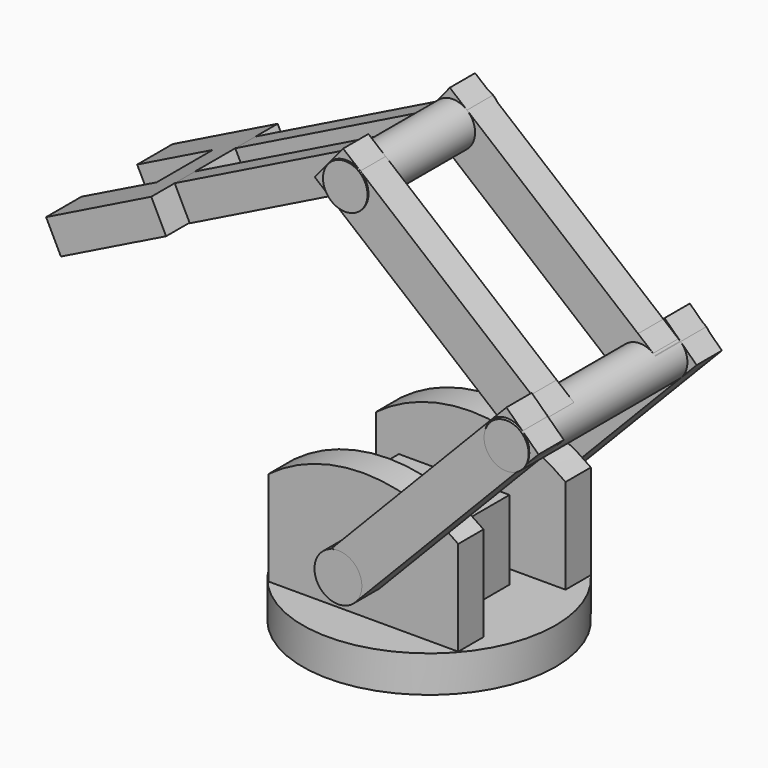
from build123d import *

# Parameters (mm, degrees)
F0_R           = 50.8
F1_DEPTH       = 14.69634
F2_W           = 76.2
F2_H           = 12.7
F3_DEPTH       = 38.1
F5_DEPTH       = 12.7
F7_DEPTH       = 12.7
F8_W           = 44.45
F8_H           = 25.4
F9_DEPTH       = 31.75
F10_R          = 9.525
F11_DEPTH      = 68.24913
F12_R          = 9.525
F13_DEPTH      = 66.70077
F14_R          = 9.525
F15_DEPTH      = 12.7
F16_R          = 9.525
F17_DEPTH      = 12.7
F19_DEPTH      = 12.7
F21_R          = 8.9662
F22_DEPTH      = 79.74323
F22_DEPTH_BACK = 12.92457
F24_DEPTH      = 12.7
F26_R          = 8.9540969
F27_DEPTH      = 54.0361
F27_DEPTH_BACK = 13.11087
F29_DEPTH      = 10.16
F31_W          = 13.2109493386
F31_H          = 63.5
F32_DEPTH      = 13.44194
F34_DEPTH      = 13.41844
F35_W          = 33.9267599266
F35_H          = 17.78
F36_DEPTH      = 13.32265
F37_R          = 8.9662
F38_DEPTH      = 12.7
F39_R          = 8.9662
F40_DEPTH      = 12.7
F41_R          = 8.9540969
F42_DEPTH      = 12.7
F43_R          = 8.9540969
F44_DEPTH      = 12.7


# Not quite as in the source:
# - a feature names something its author has since deleted; it is built from what else it names


with BuildPart() as f1:
    # F0 (on Top) → F1 (new body)
    with BuildSketch(Plane.XY):
        with Locations((78.1534910202, 35.6075726449)):
            Circle(F0_R)
    extrude(amount=F1_DEPTH)

    # F2 (on face) → F3 (join)
    with BuildSketch(Plane.XY.offset(14.69634)):
        with Locations((78.1534910202, 8.9485988323)):
            Rectangle(F2_W, F2_H)
        with Locations((78.1534910202, 62.8586142955)):
            Rectangle(F2_W, F2_H)
    extrude(amount=F3_DEPTH)

    # F4 (on face) → F5 (join)
    with BuildSketch(Plane.XZ.offset(-2.5985988323)):
        with BuildLine():
            Line((40.0534910202, 52.79634), (116.2534910202, 52.79634))
            ThreePointArc((116.2534910202, 52.79634), (78.1534910202, 65.49634), (40.0534910202, 52.79634))
        make_face()
    extrude(amount=-F5_DEPTH)

    # F6 (on face) → F7 (join)
    with BuildSketch(Plane.XZ.offset(-56.5086142955)):
        with BuildLine():
            Line((40.0534910202, 52.79634), (116.2534910202, 52.79634))
            ThreePointArc((116.2534910202, 52.79634), (78.1534910202, 65.49634), (40.0534910202, 52.79634))
        make_face()
    extrude(amount=-F7_DEPTH)

    # F8 (on face) → F9 (join)
    with BuildSketch(Plane.XY.offset(14.69634)):
        with Locations((78.1534910202, 35.4908860509)):
            Rectangle(F8_W, F8_H)
    extrude(amount=F9_DEPTH)

    # F10 (on face) → F11 (cut)
    with BuildSketch(Plane.XZ.offset(-2.5985988323)):
        with Locations((78.1534910202, 33.74634)):
            Circle(F10_R)
    extrude(amount=-F11_DEPTH, mode=Mode.SUBTRACT)


with BuildPart() as f13:
    # F12 (on face) → F13 (new body)
    with BuildSketch(Plane.XZ.offset(-2.5985988323)):
        with Locations((78.1534910202, 33.74634)):
            Circle(F12_R)
    extrude(amount=-F13_DEPTH)

    # F14 (on face) → F15 (join)
    with BuildSketch(Plane.XZ.offset(-2.5985988323)):
        with Locations((78.1534910202, 33.74634)):
            Circle(F14_R)
    extrude(amount=F15_DEPTH)

    # F16 (on face) → F17 (join)
    with BuildSketch(Plane(origin=(0, 69.2993688323, 0), x_dir=(-1, 0, 0), z_dir=(0, 1, 0))):
        with Locations((-78.1534910202, 33.74634)):
            Circle(F16_R)
    extrude(amount=F17_DEPTH)


with BuildPart() as f19:
    # F18 (on face) → F19 (new body)
    with BuildSketch(Plane.XZ.offset(-2.5985988323)):
        with BuildLine():
            Line((145.7822117796, 115.867993462), (94.9363889392, 63.238354479))
            ThreePointArc((94.9363889392, 63.238354479), (103.9505756834, 60.0201318692), (112.3786539474, 55.4836115944))
            Line((112.3786539474, 55.4836115944), (158.6790101463, 103.4083160324))
            Line((158.6790101463, 103.4083160324), (145.7822117796, 115.867993462))
        make_face()
        with BuildLine():
            Line((94.9363889392, 63.238354479), (75.1891385244, 42.7983143305))
            ThreePointArc((75.1891385244, 42.7983143305), (83.7432212229, 41.4587028845), (87.6784910202, 33.74634))
            ThreePointArc((87.6784910202, 33.74634), (87.0779374466, 30.4176944823), (85.3520068243, 27.5087927883))
            Line((85.3520068243, 27.5087927883), (112.3786539474, 55.4836115944))
            ThreePointArc((112.3786539474, 55.4836115944), (103.9505756834, 60.0201318692), (94.9363889392, 63.238354479))
        make_face()
    extrude(amount=F19_DEPTH)


with BuildPart() as f20_1:
    # F20: copy of F19
    add(f19.part.moved(Location((0, 79.43989, -0.67967))))

    # F39 (on face) → F40 (cut)
    with BuildSketch(Plane(origin=(0, 82.0384888323, 0), x_dir=(-1, 0, 0), z_dir=(0, 1, 0))):
        with Locations((-146.0007722482, 102.5100855638)):
            Circle(F39_R)
    extrude(amount=-F40_DEPTH, mode=Mode.SUBTRACT)


with BuildPart() as f22:
    # F21 (on face) → F22 (new body, two sides)
    with BuildSketch(Plane.XZ.offset(-69.3384888323)) as f22_sk:
        with Locations((146.0007722482, 102.5100855638)):
            Circle(F21_R)
    extrude(amount=F22_DEPTH)
    extrude(f22_sk.sketch, amount=-F22_DEPTH_BACK)


with BuildPart() as f24:
    # F23 (on face) → F24 (new body)
    with BuildSketch(Plane.XZ.offset(-69.3384888323)):
        Polygon((58.2396076903, 163.2934401453), (132.8123130568, 101.7634037873), (145.2934127821, 114.6823760047), (69.6369095731, 177.1066553746), align=None)
        with BuildLine():
            Line((132.8123130568, 101.7634037873), (140.8333090802, 95.1452695179))
            ThreePointArc((140.8333090802, 95.1452695179), (139.625352407, 107.7505280739), (152.230610963, 108.9584847472))
            Line((152.230610963, 108.9584847472), (145.2934127821, 114.6823760047))
            Line((145.2934127821, 114.6823760047), (132.8123130568, 101.7634037873))
        make_face()
    extrude(amount=F24_DEPTH)


with BuildPart() as f25_1:
    # F25: copy of F24
    add(f24.part.moved(Location((0, -53.58946, 0.24325))))

    # F41 (on face) → F42 (cut)
    with BuildSketch(Plane.XZ.offset(-3.0490288323)):
        with Locations((70.8448662464, 164.7446468185)):
            Circle(F41_R)
    extrude(amount=-F42_DEPTH, mode=Mode.SUBTRACT)


with BuildPart() as f27:
    # F26 (on face) → F27 (new body, two sides)
    with BuildSketch(Plane.XZ.offset(-56.6384888323)) as f27_sk:
        with Locations((70.8448662464, 164.5013968185)):
            Circle(F26_R)
    extrude(amount=F27_DEPTH)
    extrude(f27_sk.sketch, amount=-F27_DEPTH_BACK)


with BuildPart() as f29:
    # F28 (on face) → F29 (new body)
    with BuildSketch(Plane.XZ.offset(-56.6384888323)):
        with BuildLine():
            Line((-2.5902629835, 122.1002609634), (66.3009076361, 156.2517956781))
            ThreePointArc((66.3009076361, 156.2517956781), (62.113727542, 164.2841962748), (67.0794000886, 171.8600812163))
            Line((67.0794000886, 171.8600812163), (-8.6478248157, 134.319697929))
            Line((-8.6478248157, 134.319697929), (-2.5902629835, 122.1002609634))
        make_face()
    extrude(amount=F29_DEPTH)


with BuildPart() as f30_1:
    # F30: copy of F29
    add(f29.part.moved(Location((0, -30.42229, 0))))


with BuildPart() as f32:
    # F31 (on face) → F32 (new body)
    with BuildSketch(Plane(origin=(-55.1569222191, 0, 111.2636656358), x_dir=(0.8959516474, 0, 0.4441516019), z_dir=(-0.4441516019, 0, 0.8959516474))):
        with Locations((45.5043371767, 36.0230419319)):
            Rectangle(F31_W, F31_H)
    extrude(amount=-F32_DEPTH)

    # F33 (on face) → F34 (join)
    with BuildSketch(Plane(origin=(-55.1569222191, 0, 111.2636656358), x_dir=(0.8959516474, 0, 0.4441516019), z_dir=(-0.4441516019, 0, 0.8959516474))):
        Polygon((38.8988625074, 4.2730419319), (38.8988625074, 21.7697144404), (4.9334512876, 22.0530419319), (4.9334512876, 4.2730419319), align=None)
    extrude(amount=-F34_DEPTH)

    # F35 (on face) → F36 (join)
    with BuildSketch(Plane(origin=(-55.1569222191, 0, 111.2636656358), x_dir=(0.8959516474, 0, 0.4441516019), z_dir=(-0.4441516019, 0, 0.8959516474))):
        with Locations((21.9354825441, 58.8830419319)):
            Rectangle(F35_W, F35_H)
    extrude(amount=-F36_DEPTH)


with BuildPart() as f19_1:
    add(f19.part)

    # F37 (on face) → F38 (cut)
    with BuildSketch(Plane.XZ.offset(10.1014011677)):
        with Locations((146.0007722482, 103.1897555638)):
            Circle(F37_R)
    extrude(amount=-F38_DEPTH, mode=Mode.SUBTRACT)


with BuildPart() as f24_1:
    add(f24.part)

    # F43 (on face) → F44 (cut)
    with BuildSketch(Plane(origin=(0, 69.3384888323, 0), x_dir=(-1, 0, 0), z_dir=(0, 1, 0))):
        with Locations((-70.8448662464, 164.5013968185)):
            Circle(F43_R)
    extrude(amount=-F44_DEPTH, mode=Mode.SUBTRACT)


solid = Compound([f1.part, f13.part, f20_1.part, f22.part, f25_1.part, f27.part, f29.part, f30_1.part, f32.part, f19_1.part, f24_1.part])
